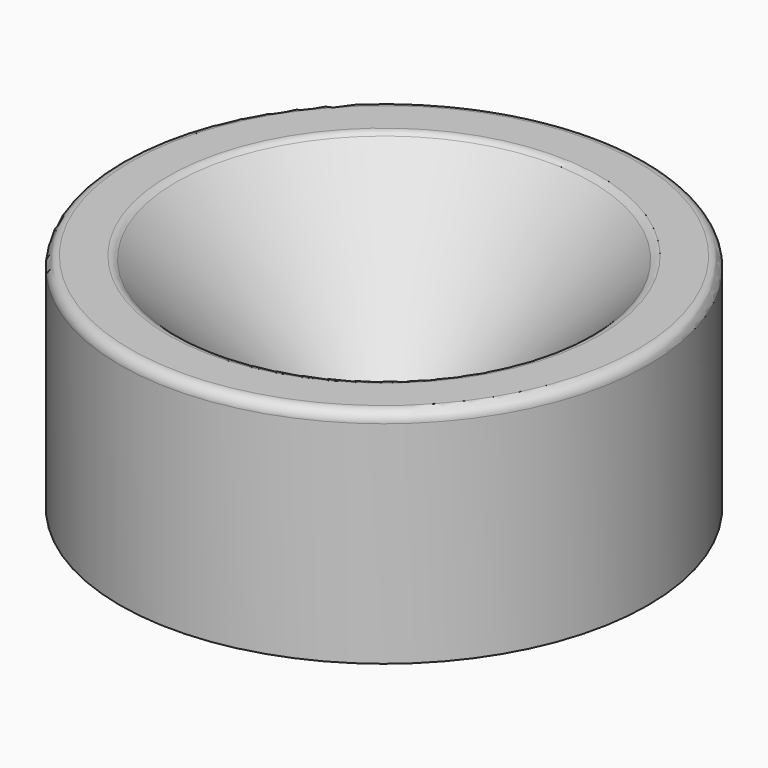
from build123d import *

# Parameters (mm, degrees)
F2_R = 0.5


with BuildPart() as f1:
    # F0 (on Front) → F1 (revolve)
    with BuildSketch(Plane.XZ):
        Polygon((10, 10.5), (2.5, 3), (2.5, 0), (12.5, 0), (12.5, 10.5), align=None)
    revolve(axis=Axis((0, 0, 15.3351295739), (0, 0, -1)))

    # F2
    f2_edges = [f1.edges().sort_by_distance(p)[0] for p in [
        (-12.5, 0, 10.5),
        (-10, 0, 10.5),
        (-2.5, 0, 3),
        (-2.5, 0, 0),
    ]]
    fillet(f2_edges, radius=F2_R)


solid = f1.part
